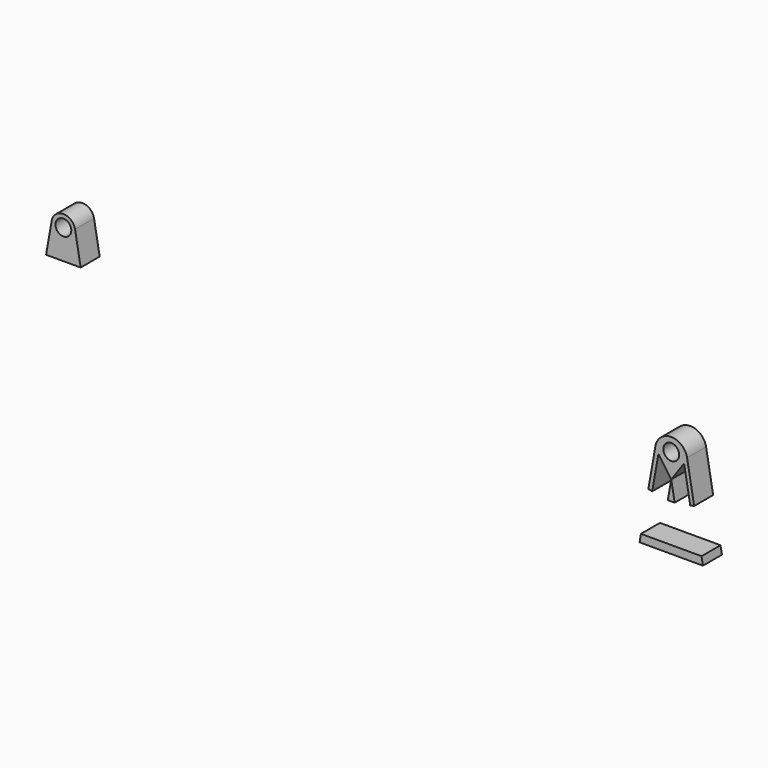
from build123d import *

# Parameters (mm, degrees)
F1_R     = 25.4
F2_DEPTH = 76.2


with BuildPart() as f2:
    # F1 (on Front) → F2 (new body)
    with BuildSketch(Plane.XZ):
        with BuildLine():
            ThreePointArc((1182.7422758102, 616.9652833939), (1220.8422758102, 578.8652833939), (1258.9422758102, 616.9652833939))
            ThreePointArc((1258.9422758102, 616.9652833939), (1220.8422758102, 655.0652833939), (1182.7422758102, 616.9652833939))
        make_face()
        with Locations((1220.8422758102, 616.9652833939)):
            Circle(F1_R, mode=Mode.SUBTRACT)
        with BuildLine():
            ThreePointArc((1182.7422758102, 616.9652833939), (1220.8422758102, 655.0652833939), (1258.9422758102, 616.9652833939))
            Line((1258.9422758102, 616.9652833939), (1271.6422758102, 616.9652833939))
            ThreePointArc((1271.6422758102, 616.9652833939), (1220.8422758102, 659.5915446577), (1170.0422758102, 616.9652833939))
            Line((1170.0422758102, 616.9652833939), (1182.7422758102, 616.9652833939))
        make_face()
        with BuildLine():
            Line((1271.6422758102, 616.9652833939), (1258.9422758102, 616.9652833939))
            ThreePointArc((1258.9422758102, 616.9652833939), (1220.8422758102, 578.8652833939), (1182.7422758102, 616.9652833939))
            Line((1182.7422758102, 616.9652833939), (1170.0422758102, 616.9652833939))
            Line((1170.0422758102, 616.9652833939), (1147.3536941437, 488.2919426757))
            Line((1147.3536941437, 488.2919426757), (1159.860752607, 486.0866108193))
            Line((1159.860752607, 486.0866108193), (1179.6353693827, 598.2340354293))
            Line((1179.6353693827, 598.2340354293), (1220.8422758102, 539.3844741508))
            Line((1220.8422758102, 539.3844741508), (1262.0491822378, 598.2340354293))
            Line((1262.0491822378, 598.2340354293), (1281.8237990135, 486.0866108193))
            Line((1281.8237990135, 486.0866108193), (1294.3308574767, 488.2919426757))
            Line((1294.3308574767, 488.2919426757), (1271.6422758102, 616.9652833939))
        make_face()
    extrude(amount=F2_DEPTH)


with BuildPart() as f2b:
    # F1 (on Front) → F2, piece 2 (new body)
    with BuildSketch(Plane.XZ):
        Polygon((1317.9635705002, 354.2641669573), (1305.0676525293, 354.2641669573), (1309.5463578393, 328.8641669573), (1322.4422758102, 328.8641669573), align=None)
        Polygon((1309.5463578393, 328.8641669573), (1305.0676525293, 354.2641669573), (1253.4839806455, 354.2641669573), (1257.9626859555, 328.8641669573), align=None)
        Polygon((1188.200570975, 354.2641669573), (1136.6168990912, 354.2641669573), (1132.1381937812, 328.8641669573), (1183.721865665, 328.8641669573), align=None)
        Polygon((1132.1381937812, 328.8641669573), (1136.6168990912, 354.2641669573), (1123.7209811202, 354.2641669573), (1119.2422758102, 328.8641669573), align=None)
        Polygon((1257.9626859555, 328.8641669573), (1253.4839806455, 354.2641669573), (1188.200570975, 354.2641669573), (1183.721865665, 328.8641669573), align=None)
    extrude(amount=F2_DEPTH)


with BuildPart() as f2c:
    # F1 (on Front) → F2, piece 3 (new body)
    with BuildSketch(Plane.XZ):
        Polygon((1209.88898646, 477.2652833939), (1231.7955651605, 477.2652833939), (1220.8422758102, 539.3844741508), align=None)
    extrude(amount=F2_DEPTH)


with BuildPart() as f2d:
    # F1 (on Front) → F2, piece 4 (new body)
    with BuildSketch(Plane.XZ):
        with BuildLine():
            ThreePointArc((-766.8345454561, 623.581278963), (-732.634003865, 579.0102653966), (-691.2133700663, 616.9652833939))
            ThreePointArc((-691.2133700663, 616.9652833939), (-691.358352069, 620.2859171925), (-691.7921946765, 623.581278963))
            ThreePointArc((-691.7921946765, 623.581278963), (-729.3133700663, 655.0652833939), (-766.8345454561, 623.581278963))
        make_face()
        with Locations((-729.3133700663, 616.9652833939)):
            Circle(F1_R, mode=Mode.SUBTRACT)
        with BuildLine():
            ThreePointArc((-691.7921946765, 623.581278963), (-691.358352069, 620.2859171925), (-691.2133700663, 616.9652833939))
            ThreePointArc((-691.2133700663, 616.9652833939), (-732.634003865, 579.0102653966), (-766.8345454561, 623.581278963))
            Line((-766.8345454561, 623.581278963), (-784.7962688916, 521.7152833939))
            Line((-784.7962688916, 521.7152833939), (-673.830471241, 521.7152833939))
            Line((-673.830471241, 521.7152833939), (-691.7921946765, 623.581278963))
        make_face()
    extrude(amount=F2_DEPTH)


solid = Compound([f2.part, f2b.part, f2c.part, f2d.part])
